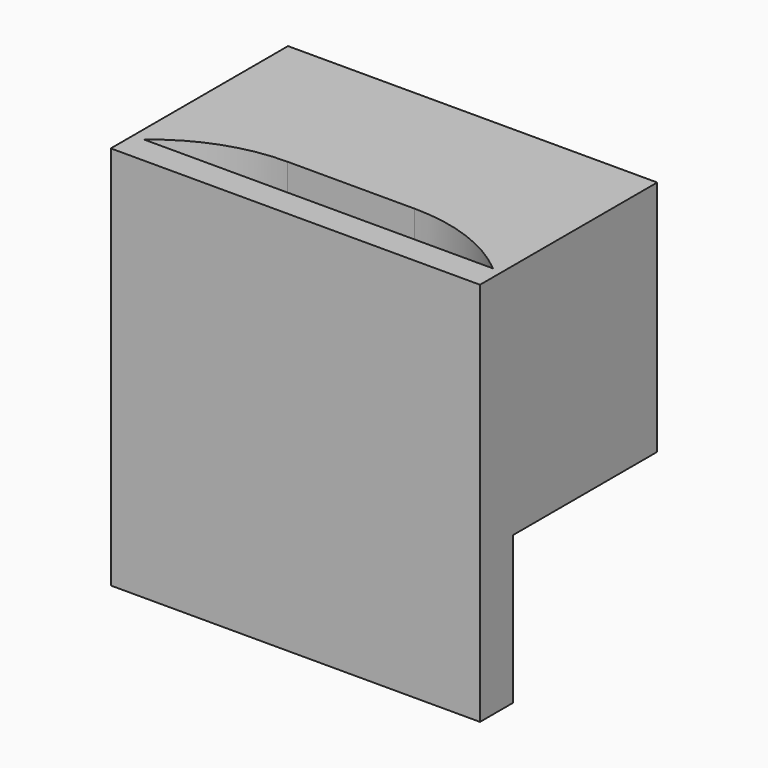
from build123d import *

# Parameters (mm, degrees)
F0_W         = 63.5
F0_H         = 63.5
F1_DEPTH     = 38.1
F2_DEPTH     = 58.42
F3_W         = 60
F3_H         = 7
F4_DEPTH     = 38.1
F5_W         = 60
F5_H         = 19.05
F6_DEPTH     = 50.8
F7_DEPTH     = 25.4
F8_W         = 38.1
F8_H         = 17.6288653165
F9_DEPTH     = 76.2
F10_T1_DEPTH = 19.05
F11_W        = 63.5
F11_H        = 13.4413276523
F12_DEPTH    = 25.4
F13_DEPTH    = 6.35


# Not quite as in the source:
# - a fillet or chamfer that OpenCascade refuses, or shapes differently, is made with other operations: its cross-section is extruded or revolved along the edge and cut away or added


with BuildPart() as f1:
    # F0 (on Top) → F1 (new body)
    with BuildSketch(Plane.XY):
        with Locations((-0.7267157435, 4.9544320554)):
            Rectangle(F0_W, F0_H)
    extrude(amount=F1_DEPTH)

    # F0 (on Top) → F2 (join)
    with BuildSketch(Plane.XY):
        with Locations((-0.7267157435, 4.9544320554)):
            Rectangle(F0_W, F0_H)
    extrude(amount=F2_DEPTH)

    # F3 (on face) → F4 (cut)
    with BuildSketch(Plane.XY.offset(58.42)):
        with Locations((-0.5849367008, 6.9008102814)):
            Rectangle(F3_W, F3_H)
    extrude(amount=-F4_DEPTH, mode=Mode.SUBTRACT)

    # F5 (on face) → F6 (cut)
    with BuildSketch(Plane.XZ.offset(-10.4008102814)):
        with Locations((-0.5849367008, 29.845)):
            Rectangle(F5_W, F5_H)
    extrude(amount=-F6_DEPTH, mode=Mode.SUBTRACT)

    # F7 (cut): a face of the model
    f7_faces = [f1.faces().sort_by_distance(p)[0] for p in [
        (-0.7267157435, -26.7955679446, 29.21),
    ]]
    extrude(f7_faces, amount=-F7_DEPTH, mode=Mode.SUBTRACT)

    # F8 (on face) → F9 (cut)
    with BuildSketch(Plane.YZ.offset(31.0232842565)):
        with Locations((17.6544320554, 8.8144326583)):
            Rectangle(F8_W, F8_H)
    extrude(amount=-F9_DEPTH, mode=Mode.SUBTRACT)

    # F10: fillet of radius 29.4340917525 on 2 edges, made by hand

    # F10_s2 → F10_t1 (join)
    with BuildSketch(Plane.XY.offset(39.37)):
        with BuildLine():
            ThreePointArc((29.4150632992, 3.4008102814), (20.5103197353, 8.5954433667), (10.3604763309, 10.4008102814))
            Line((10.3604763309, 10.4008102814), (29.4150632992, 10.4008102814))
            Line((29.4150632992, 10.4008102814), (29.4150632992, 3.4008102814))
        make_face()
        with BuildLine():
            ThreePointArc((-30.5849367008, 3.4008102814), (-21.6801931368, 8.5954433667), (-11.5303497324, 10.4008102814))
            Line((-11.5303497324, 10.4008102814), (-30.5849367008, 10.4008102814))
            Line((-30.5849367008, 10.4008102814), (-30.5849367008, 3.4008102814))
        make_face()
    extrude(amount=F10_T1_DEPTH)

    # F11 (on face) → F12 (join)
    with BuildSketch(Plane(origin=(0, 0, 17.6288653165), x_dir=(1, 0, 0), z_dir=(0, 0, -1))):
        with Locations((-0.7267157435, -5.3250958815)):
            Rectangle(F11_W, F11_H)
    extrude(amount=F12_DEPTH)

    # F13 (cut): a face of the model
    f13_faces = [f1.faces().sort_by_distance(p)[0] for p in [
        (-0.7267157435, 12.0457597077, 4.9288653165),
    ]]
    extrude(f13_faces, amount=-F13_DEPTH, mode=Mode.SUBTRACT)


solid = f1.part
